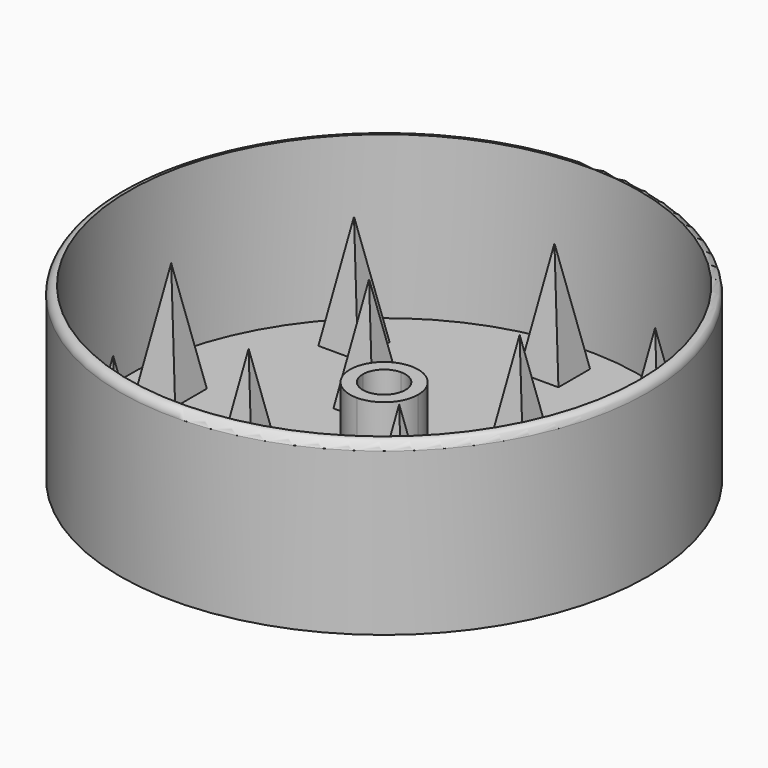
from build123d import *

# Parameters (mm, degrees)
F0_R     = 31
F0_R_2   = 30
F0_W     = 5
F0_H     = 5
F1_DEPTH = 1
F2_DEPTH = 20
F3_DEPTH = 10
F4_DEPTH = 15
F4_TAPER = 10
F5_R     = 0.99999
F6_DEPTH = 5


# Not quite as in the source:
# - a fillet or chamfer is up to 0.001 mm smaller than in the source, because OpenCascade refuses the exact size


with BuildPart() as f1:
    # F0 (on Top) → F1 (new body)
    with BuildSketch(Plane.XY):
        Circle(F0_R)
        Circle(F0_R_2, mode=Mode.SUBTRACT)
        Circle(F0_R_2)
        with Locations((-17.6776695297, -17.6776695297)):
            Rectangle(F0_W, F0_H, mode=Mode.SUBTRACT)
        Polygon((-2.5, -22.5), (0, -22.5), (2.5, -22.5), (2.5, -27.5), (-2.5, -27.5), align=None, mode=Mode.SUBTRACT)
        with Locations((17.6776695297, -17.6776695297)):
            Rectangle(F0_W, F0_H, mode=Mode.SUBTRACT)
        Polygon((-22.5, 2.5), (-22.5, 0), (-22.5, -2.5), (-27.5, -2.5), (-27.5, 2.5), align=None, mode=Mode.SUBTRACT)
        with Locations((-17.6776695297, 17.6776695297)):
            Rectangle(F0_W, F0_H, mode=Mode.SUBTRACT)
        with BuildLine():
            ThreePointArc((-15.1776695297, 15.1776695297), (-8.2140955588, 19.8305809006), (0, 21.4644660941))
            ThreePointArc((0, 21.4644660941), (8.2140955588, 19.8305809006), (15.1776695297, 15.1776695297))
            ThreePointArc((15.1776695297, 15.1776695297), (19.8305809006, 8.2140955588), (21.4644660941, 0))
            ThreePointArc((21.4644660941, 0), (19.8305809006, -8.2140955588), (15.1776695297, -15.1776695297))
            ThreePointArc((15.1776695297, -15.1776695297), (8.2140955588, -19.8305809006), (0, -21.4644660941))
            ThreePointArc((0, -21.4644660941), (-8.2140955588, -19.8305809006), (-15.1776695297, -15.1776695297))
            ThreePointArc((-15.1776695297, -15.1776695297), (-19.8305809006, -8.2140955588), (-21.4644660941, 0))
            ThreePointArc((-21.4644660941, 0), (-19.8305809006, 8.2140955588), (-15.1776695297, 15.1776695297))
        make_face(mode=Mode.SUBTRACT)
        Polygon((22.5, -2.5), (22.5, 0), (22.5, 2.5), (27.5, 2.5), (27.5, -2.5), align=None, mode=Mode.SUBTRACT)
        Polygon((2.5, 22.5), (0, 22.5), (-2.5, 22.5), (-2.5, 27.5), (2.5, 27.5), align=None, mode=Mode.SUBTRACT)
        with Locations((17.6776695297, 17.6776695297)):
            Rectangle(F0_W, F0_H, mode=Mode.SUBTRACT)
        with BuildLine():
            Line((0, 21.4644660941), (0, 12.5))
            ThreePointArc((0, 12.5), (3.2848701936, 12.0606644847), (6.3388347648, 10.7735404498))
            Line((6.3388347648, 10.7735404498), (6.3388347648, 11.3388347648))
            Line((6.3388347648, 11.3388347648), (11.3388347648, 11.3388347648))
            Line((11.3388347648, 11.3388347648), (15.1776695297, 15.1776695297))
            ThreePointArc((15.1776695297, 15.1776695297), (8.2140955588, 19.8305809006), (0, 21.4644660941))
        make_face()
        with BuildLine():
            ThreePointArc((10.7735404498, 6.3388347648), (12.0606644847, 3.2848701936), (12.5, 0))
            Line((12.5, 0), (21.4644660941, 0))
            ThreePointArc((21.4644660941, 0), (19.8305809006, 8.2140955588), (15.1776695297, 15.1776695297))
            Line((15.1776695297, 15.1776695297), (11.3388347648, 11.3388347648))
            Line((11.3388347648, 11.3388347648), (11.3388347648, 6.3388347648))
            Line((11.3388347648, 6.3388347648), (10.7735404498, 6.3388347648))
        make_face()
        with BuildLine():
            ThreePointArc((6.3388347648, -10.7735404498), (3.2848701936, -12.0606644847), (0, -12.5))
            Line((0, -12.5), (0, -21.4644660941))
            ThreePointArc((0, -21.4644660941), (8.2140955588, -19.8305809006), (15.1776695297, -15.1776695297))
            ThreePointArc((15.1776695297, -15.1776695297), (19.8305809006, -8.2140955588), (21.4644660941, 0))
            Line((21.4644660941, 0), (12.5, 0))
            ThreePointArc((12.5, 0), (12.0606644847, -3.2848701936), (10.7735404498, -6.3388347648))
            Line((10.7735404498, -6.3388347648), (11.3388347648, -6.3388347648))
            Line((11.3388347648, -6.3388347648), (11.3388347648, -11.3388347648))
            Line((11.3388347648, -11.3388347648), (6.3388347648, -11.3388347648))
            Line((6.3388347648, -11.3388347648), (6.3388347648, -10.7735404498))
        make_face()
        with BuildLine():
            Line((0, -21.4644660941), (0, -12.5))
            ThreePointArc((0, -12.5), (-3.2848701936, -12.0606644847), (-6.3388347648, -10.7735404498))
            Line((-6.3388347648, -10.7735404498), (-6.3388347648, -11.3388347648))
            Line((-6.3388347648, -11.3388347648), (-11.3388347648, -11.3388347648))
            Line((-11.3388347648, -11.3388347648), (-11.3388347648, -6.3388347648))
            Line((-11.3388347648, -6.3388347648), (-10.7735404498, -6.3388347648))
            ThreePointArc((-10.7735404498, -6.3388347648), (-12.0606644847, -3.2848701936), (-12.5, 0))
            Line((-12.5, 0), (-21.4644660941, 0))
            ThreePointArc((-21.4644660941, 0), (-19.8305809006, -8.2140955588), (-15.1776695297, -15.1776695297))
            ThreePointArc((-15.1776695297, -15.1776695297), (-8.2140955588, -19.8305809006), (0, -21.4644660941))
        make_face()
        with BuildLine():
            ThreePointArc((-6.3388347648, 10.7735404498), (-3.2848701936, 12.0606644847), (0, 12.5))
            Line((0, 12.5), (0, 21.4644660941))
            ThreePointArc((0, 21.4644660941), (-8.2140955588, 19.8305809006), (-15.1776695297, 15.1776695297))
            ThreePointArc((-15.1776695297, 15.1776695297), (-19.8305809006, 8.2140955588), (-21.4644660941, 0))
            Line((-21.4644660941, 0), (-12.5, 0))
            ThreePointArc((-12.5, 0), (-12.0606644847, 3.2848701936), (-10.7735404498, 6.3388347648))
            Line((-10.7735404498, 6.3388347648), (-11.3388347648, 6.3388347648))
            Line((-11.3388347648, 6.3388347648), (-11.3388347648, 11.3388347648))
            Line((-11.3388347648, 11.3388347648), (-6.3388347648, 11.3388347648))
            Line((-6.3388347648, 11.3388347648), (-6.3388347648, 10.7735404498))
        make_face()
        with BuildLine():
            Line((0, 12.5), (0, 4))
            ThreePointArc((0, 4), (1.5307337295, 3.69551813), (2.8284271247, 2.8284271247))
            Line((2.8284271247, 2.8284271247), (6.3388347648, 6.3388347648))
            Line((6.3388347648, 6.3388347648), (6.3388347648, 10.7735404498))
            ThreePointArc((6.3388347648, 10.7735404498), (3.2848701936, 12.0606644847), (0, 12.5))
        make_face()
        with BuildLine():
            ThreePointArc((-4, 0), (-2.8284271247, 2.8284271247), (0, 4))
            Line((0, 4), (0, 12.5))
            ThreePointArc((0, 12.5), (-3.2848701936, 12.0606644847), (-6.3388347648, 10.7735404498))
            Line((-6.3388347648, 10.7735404498), (-6.3388347648, 6.3388347648))
            Line((-6.3388347648, 6.3388347648), (-10.7735404498, 6.3388347648))
            ThreePointArc((-10.7735404498, 6.3388347648), (-12.0606644847, 3.2848701936), (-12.5, 0))
            Line((-12.5, 0), (-4, 0))
        make_face()
        with BuildLine():
            ThreePointArc((2.8284271247, 2.8284271247), (3.69551813, 1.5307337295), (4, 0))
            Line((4, 0), (12.5, 0))
            ThreePointArc((12.5, 0), (12.0606644847, 3.2848701936), (10.7735404498, 6.3388347648))
            Line((10.7735404498, 6.3388347648), (6.3388347648, 6.3388347648))
            Line((6.3388347648, 6.3388347648), (2.8284271247, 2.8284271247))
        make_face()
        with BuildLine():
            ThreePointArc((4, 0), (2.8284271247, -2.8284271247), (0, -4))
            Line((0, -4), (0, -12.5))
            ThreePointArc((0, -12.5), (3.2848701936, -12.0606644847), (6.3388347648, -10.7735404498))
            Line((6.3388347648, -10.7735404498), (6.3388347648, -6.3388347648))
            Line((6.3388347648, -6.3388347648), (10.7735404498, -6.3388347648))
            ThreePointArc((10.7735404498, -6.3388347648), (12.0606644847, -3.2848701936), (12.5, 0))
            Line((12.5, 0), (4, 0))
        make_face()
        with BuildLine():
            Line((0, -12.5), (0, -4))
            ThreePointArc((0, -4), (-2.8284271247, -2.8284271247), (-4, 0))
            Line((-4, 0), (-12.5, 0))
            ThreePointArc((-12.5, 0), (-12.0606644847, -3.2848701936), (-10.7735404498, -6.3388347648))
            Line((-10.7735404498, -6.3388347648), (-6.3388347648, -6.3388347648))
            Line((-6.3388347648, -6.3388347648), (-6.3388347648, -10.7735404498))
            ThreePointArc((-6.3388347648, -10.7735404498), (-3.2848701936, -12.0606644847), (0, -12.5))
        make_face()
        Polygon((22.5, 2.5), (25, 0), (27.5, 2.5), align=None)
        Polygon((27.5, 2.5), (25, 0), (27.5, -2.5), align=None)
        Polygon((27.5, -2.5), (25, 0), (22.5, -2.5), align=None)
        Polygon((25, 0), (22.5, 0), (22.5, -2.5), align=None)
        Polygon((22.5, 2.5), (22.5, 0), (25, 0), align=None)
        Polygon((17.6776695297, 17.6776695297), (15.1776695297, 15.1776695297), (20.1776695297, 15.1776695297), align=None)
        Polygon((15.1776695297, 20.1776695297), (17.6776695297, 17.6776695297), (20.1776695297, 20.1776695297), align=None)
        Polygon((20.1776695297, 20.1776695297), (17.6776695297, 17.6776695297), (20.1776695297, 15.1776695297), align=None)
        Polygon((15.1776695297, 20.1776695297), (15.1776695297, 15.1776695297), (17.6776695297, 17.6776695297), align=None)
        Polygon((-2.5, 27.5), (0, 25), (2.5, 27.5), align=None)
        Polygon((2.5, 27.5), (0, 25), (2.5, 22.5), align=None)
        Polygon((-2.5, 22.5), (0, 22.5), (0, 25), align=None)
        Polygon((0, 25), (0, 22.5), (2.5, 22.5), align=None)
        Polygon((-2.5, 22.5), (0, 25), (-2.5, 27.5), align=None)
        Polygon((-17.6776695297, 17.6776695297), (-15.1776695297, 20.1776695297), (-20.1776695297, 20.1776695297), align=None)
        Polygon((-17.6776695297, 17.6776695297), (-15.1776695297, 15.1776695297), (-15.1776695297, 20.1776695297), align=None)
        Polygon((-20.1776695297, 15.1776695297), (-15.1776695297, 15.1776695297), (-17.6776695297, 17.6776695297), align=None)
        Polygon((-20.1776695297, 20.1776695297), (-20.1776695297, 15.1776695297), (-17.6776695297, 17.6776695297), align=None)
        Polygon((-8.8388347762, 8.8388347535), (-6.3388347648, 11.3388347648), (-11.3388347648, 11.3388347648), align=None)
        Polygon((-11.3388347648, 6.3388347648), (-8.8388347762, 8.8388347535), (-11.3388347648, 11.3388347648), align=None)
        with BuildLine():
            ThreePointArc((-8.8388347762, 8.8388347535), (-9.8855356702, 7.650240814), (-10.7735404498, 6.3388347648))
            Line((-10.7735404498, 6.3388347648), (-6.3388347648, 6.3388347648))
            Line((-6.3388347648, 6.3388347648), (-8.8388347648, 8.8388347648))
        make_face()
        with BuildLine():
            Line((-6.3388347648, 6.3388347648), (-6.3388347648, 10.7735404498))
            ThreePointArc((-6.3388347648, 10.7735404498), (-7.6502408267, 9.8855356604), (-8.8388347762, 8.8388347535))
            Line((-8.8388347648, 8.8388347648), (-6.3388347648, 6.3388347648))
        make_face()
        with BuildLine():
            Line((6.3388347648, 10.7735404498), (6.3388347648, 6.3388347648))
            Line((6.3388347648, 6.3388347648), (8.8388347648, 8.8388347648))
            ThreePointArc((8.8388347535, 8.8388347762), (7.650240814, 9.8855356702), (6.3388347648, 10.7735404498))
        make_face()
        Polygon((6.3388347648, 11.3388347648), (8.8388347535, 8.8388347762), (11.3388347648, 11.3388347648), align=None)
        Polygon((11.3388347648, 11.3388347648), (8.8388347648, 8.8388347648), (11.3388347648, 6.3388347648), align=None)
        with BuildLine():
            Line((8.8388347648, 8.8388347648), (6.3388347648, 6.3388347648))
            Line((6.3388347648, 6.3388347648), (10.7735404498, 6.3388347648))
            ThreePointArc((10.7735404498, 6.3388347648), (9.8855356604, 7.6502408267), (8.8388347535, 8.8388347762))
        make_face()
        with BuildLine():
            ThreePointArc((8.8388347578, -8.8388347719), (9.8855356623, -7.6502408243), (10.7735404498, -6.3388347648))
            Line((10.7735404498, -6.3388347648), (6.3388347648, -6.3388347648))
            Line((6.3388347648, -6.3388347648), (8.8388347648, -8.8388347648))
        make_face()
        Polygon((11.3388347648, -6.3388347648), (8.8388347578, -8.8388347719), (11.3388347648, -11.3388347648), align=None)
        Polygon((8.8388347578, -8.8388347719), (6.3388347648, -11.3388347648), (11.3388347648, -11.3388347648), align=None)
        with BuildLine():
            Line((6.3388347648, -6.3388347648), (6.3388347648, -10.7735404498))
            ThreePointArc((6.3388347648, -10.7735404498), (7.6502408164, -9.8855356684), (8.8388347578, -8.8388347719))
            Line((8.8388347648, -8.8388347648), (6.3388347648, -6.3388347648))
        make_face()
        with BuildLine():
            Line((-6.3388347648, -6.3388347648), (-10.7735404498, -6.3388347648))
            ThreePointArc((-10.7735404498, -6.3388347648), (-9.8855356524, -7.650240837), (-8.838834735, -8.8388347946))
            Line((-8.8388347648, -8.8388347648), (-6.3388347648, -6.3388347648))
        make_face()
        with BuildLine():
            ThreePointArc((-8.838834735, -8.8388347946), (-7.6502408037, -9.8855356782), (-6.3388347648, -10.7735404498))
            Line((-6.3388347648, -10.7735404498), (-6.3388347648, -6.3388347648))
            Line((-6.3388347648, -6.3388347648), (-8.8388347648, -8.8388347648))
        make_face()
        Polygon((-11.3388347648, -11.3388347648), (-6.3388347648, -11.3388347648), (-8.838834735, -8.8388347946), align=None)
        Polygon((-27.5, 2.5), (-25, 0), (-22.5, 2.5), align=None)
        Polygon((-25, 0), (-22.5, 0), (-22.5, 2.5), align=None)
        Polygon((-22.5, -2.5), (-22.5, 0), (-25, 0), align=None)
        Polygon((-22.5, -2.5), (-25, 0), (-27.5, -2.5), align=None)
        Polygon((-27.5, -2.5), (-25, 0), (-27.5, 2.5), align=None)
        with BuildLine():
            ThreePointArc((-2.5, 0), (-1.767766953, 1.767766953), (0, 2.5))
            Line((0, 2.5), (0, 4))
            ThreePointArc((0, 4), (-2.8284271247, 2.8284271247), (-4, 0))
            Line((-4, 0), (-2.5, 0))
        make_face()
        with BuildLine():
            ThreePointArc((2.5, 0), (1.767766953, -1.767766953), (0, -2.5))
            Line((0, -2.5), (0, -4))
            ThreePointArc((0, -4), (2.8284271247, -2.8284271247), (4, 0))
            Line((4, 0), (2.5, 0))
        make_face()
        with BuildLine():
            Line((0, -4), (0, -2.5))
            ThreePointArc((0, -2.5), (-1.767766953, -1.767766953), (-2.5, 0))
            Line((-2.5, 0), (-4, 0))
            ThreePointArc((-4, 0), (-2.8284271247, -2.8284271247), (0, -4))
        make_face()
        with BuildLine():
            ThreePointArc((1.767766953, 1.767766953), (2.3096988313, 0.9567085809), (2.5, 0))
            Line((2.5, 0), (4, 0))
            ThreePointArc((4, 0), (3.69551813, 1.5307337295), (2.8284271247, 2.8284271247))
            Line((2.8284271247, 2.8284271247), (1.767766953, 1.767766953))
        make_face()
        with BuildLine():
            Line((0, 4), (0, 2.5))
            ThreePointArc((0, 2.5), (0.9567085809, 2.3096988313), (1.767766953, 1.767766953))
            Line((1.767766953, 1.767766953), (2.8284271247, 2.8284271247))
            ThreePointArc((2.8284271247, 2.8284271247), (1.5307337295, 3.69551813), (0, 4))
        make_face()
        Polygon((-11.3388347648, -11.3388347648), (-8.8388347648, -8.8388347648), (-11.3388347648, -6.3388347648), align=None)
        Polygon((-17.6776695297, -17.6776695297), (-15.1776695297, -15.1776695297), (-20.1776695297, -15.1776695297), align=None)
        Polygon((-15.1776695297, -20.1776695297), (-15.1776695297, -15.1776695297), (-17.6776695297, -17.6776695297), align=None)
        Polygon((-20.1776695297, -20.1776695297), (-15.1776695297, -20.1776695297), (-17.6776695297, -17.6776695297), align=None)
        Polygon((-17.6776695297, -17.6776695297), (-20.1776695297, -15.1776695297), (-20.1776695297, -20.1776695297), align=None)
        Polygon((20.1776695297, -15.1776695297), (15.1776695297, -15.1776695297), (17.6776695297, -17.6776695297), align=None)
        Polygon((20.1776695297, -20.1776695297), (20.1776695297, -15.1776695297), (17.6776695297, -17.6776695297), align=None)
        Polygon((17.6776695297, -17.6776695297), (15.1776695297, -20.1776695297), (20.1776695297, -20.1776695297), align=None)
        Polygon((17.6776695297, -17.6776695297), (15.1776695297, -15.1776695297), (15.1776695297, -20.1776695297), align=None)
        Polygon((2.5, -22.5), (0, -25), (2.5, -27.5), align=None)
        Polygon((2.5, -27.5), (0, -25), (-2.5, -27.5), align=None)
        Polygon((-2.5, -27.5), (0, -25), (-2.5, -22.5), align=None)
        Polygon((0, -25), (0, -22.5), (-2.5, -22.5), align=None)
        Polygon((2.5, -22.5), (0, -22.5), (0, -25), align=None)
        with BuildLine():
            Line((11.3388347648, -6.3388347648), (10.7735404498, -6.3388347648))
            ThreePointArc((10.7735404498, -6.3388347648), (9.8855356623, -7.6502408243), (8.8388347578, -8.8388347719))
            Line((8.8388347578, -8.8388347719), (11.3388347648, -6.3388347648))
        make_face()
        with BuildLine():
            ThreePointArc((8.8388347578, -8.8388347719), (7.6502408164, -9.8855356684), (6.3388347648, -10.7735404498))
            Line((6.3388347648, -10.7735404498), (6.3388347648, -11.3388347648))
            Line((6.3388347648, -11.3388347648), (8.8388347578, -8.8388347719))
        make_face()
        with BuildLine():
            Line((-6.3388347648, -11.3388347648), (-6.3388347648, -10.7735404498))
            ThreePointArc((-6.3388347648, -10.7735404498), (-7.6502408037, -9.8855356782), (-8.838834735, -8.8388347946))
            Line((-8.838834735, -8.8388347946), (-6.3388347648, -11.3388347648))
        make_face()
        with BuildLine():
            ThreePointArc((-8.838834735, -8.8388347946), (-9.8855356524, -7.650240837), (-10.7735404498, -6.3388347648))
            Line((-10.7735404498, -6.3388347648), (-11.3388347648, -6.3388347648))
            Line((-11.3388347648, -6.3388347648), (-8.838834735, -8.8388347946))
        make_face()
        with BuildLine():
            ThreePointArc((8.8388347535, 8.8388347762), (9.8855356604, 7.6502408267), (10.7735404498, 6.3388347648))
            Line((10.7735404498, 6.3388347648), (11.3388347648, 6.3388347648))
            Line((11.3388347648, 6.3388347648), (8.8388347535, 8.8388347762))
        make_face()
        with BuildLine():
            Line((6.3388347648, 11.3388347648), (6.3388347648, 10.7735404498))
            ThreePointArc((6.3388347648, 10.7735404498), (7.650240814, 9.8855356702), (8.8388347535, 8.8388347762))
            Line((8.8388347535, 8.8388347762), (6.3388347648, 11.3388347648))
        make_face()
        with BuildLine():
            ThreePointArc((-8.8388347762, 8.8388347535), (-7.6502408267, 9.8855356604), (-6.3388347648, 10.7735404498))
            Line((-6.3388347648, 10.7735404498), (-6.3388347648, 11.3388347648))
            Line((-6.3388347648, 11.3388347648), (-8.8388347762, 8.8388347535))
        make_face()
        with BuildLine():
            Line((-11.3388347648, 6.3388347648), (-10.7735404498, 6.3388347648))
            ThreePointArc((-10.7735404498, 6.3388347648), (-9.8855356702, 7.650240814), (-8.8388347762, 8.8388347535))
            Line((-8.8388347762, 8.8388347535), (-11.3388347648, 6.3388347648))
        make_face()
        with BuildLine():
            Line((0, 2.5), (0, 0))
            Line((0, 0), (1.767766953, 1.767766953))
            ThreePointArc((1.767766953, 1.767766953), (0.9567085809, 2.3096988313), (0, 2.5))
        make_face()
        with BuildLine():
            Line((1.767766953, 1.767766953), (0, 0))
            Line((0, 0), (2.5, 0))
            ThreePointArc((2.5, 0), (2.3096988313, 0.9567085809), (1.767766953, 1.767766953))
        make_face()
        with BuildLine():
            Line((2.5, 0), (0, 0))
            Line((0, 0), (0, -2.5))
            ThreePointArc((0, -2.5), (1.767766953, -1.767766953), (2.5, 0))
        make_face()
        with BuildLine():
            Line((0, -2.5), (0, 0))
            Line((0, 0), (-2.5, 0))
            ThreePointArc((-2.5, 0), (-1.767766953, -1.767766953), (0, -2.5))
        make_face()
        with BuildLine():
            Line((-2.5, 0), (0, 0))
            Line((0, 0), (0, 2.5))
            ThreePointArc((0, 2.5), (-1.767766953, 1.767766953), (-2.5, 0))
        make_face()
    extrude(amount=F1_DEPTH)

    # F0 (on Top) → F2 (join)
    with BuildSketch(Plane.XY):
        Circle(F0_R)
        Circle(F0_R_2, mode=Mode.SUBTRACT)
    extrude(amount=F2_DEPTH)

    # F0 (on Top) → F3 (join)
    with BuildSketch(Plane.XY):
        with BuildLine():
            ThreePointArc((2.5, 0), (1.767766953, -1.767766953), (0, -2.5))
            Line((0, -2.5), (0, -4))
            ThreePointArc((0, -4), (2.8284271247, -2.8284271247), (4, 0))
            Line((4, 0), (2.5, 0))
        make_face()
        with BuildLine():
            ThreePointArc((1.767766953, 1.767766953), (2.3096988313, 0.9567085809), (2.5, 0))
            Line((2.5, 0), (4, 0))
            ThreePointArc((4, 0), (3.69551813, 1.5307337295), (2.8284271247, 2.8284271247))
            Line((2.8284271247, 2.8284271247), (1.767766953, 1.767766953))
        make_face()
        with BuildLine():
            Line((0, 4), (0, 2.5))
            ThreePointArc((0, 2.5), (0.9567085809, 2.3096988313), (1.767766953, 1.767766953))
            Line((1.767766953, 1.767766953), (2.8284271247, 2.8284271247))
            ThreePointArc((2.8284271247, 2.8284271247), (1.5307337295, 3.69551813), (0, 4))
        make_face()
        with BuildLine():
            ThreePointArc((-2.5, 0), (-1.767766953, 1.767766953), (0, 2.5))
            Line((0, 2.5), (0, 4))
            ThreePointArc((0, 4), (-2.8284271247, 2.8284271247), (-4, 0))
            Line((-4, 0), (-2.5, 0))
        make_face()
        with BuildLine():
            Line((0, -4), (0, -2.5))
            ThreePointArc((0, -2.5), (-1.767766953, -1.767766953), (-2.5, 0))
            Line((-2.5, 0), (-4, 0))
            ThreePointArc((-4, 0), (-2.8284271247, -2.8284271247), (0, -4))
        make_face()
    extrude(amount=F3_DEPTH)

    # F0 (on Top) → F4 (join)
    with BuildSketch(Plane.XY):
        Polygon((2.5, -27.5), (0, -25), (-2.5, -27.5), align=None)
        Polygon((2.5, -22.5), (0, -25), (2.5, -27.5), align=None)
        Polygon((2.5, -22.5), (0, -22.5), (0, -25), align=None)
        Polygon((0, -25), (0, -22.5), (-2.5, -22.5), align=None)
        Polygon((-2.5, -27.5), (0, -25), (-2.5, -22.5), align=None)
        Polygon((17.6776695297, -17.6776695297), (15.1776695297, -15.1776695297), (15.1776695297, -20.1776695297), align=None)
        Polygon((17.6776695297, -17.6776695297), (15.1776695297, -20.1776695297), (20.1776695297, -20.1776695297), align=None)
        Polygon((20.1776695297, -20.1776695297), (20.1776695297, -15.1776695297), (17.6776695297, -17.6776695297), align=None)
        Polygon((20.1776695297, -15.1776695297), (15.1776695297, -15.1776695297), (17.6776695297, -17.6776695297), align=None)
        Polygon((8.8388347578, -8.8388347719), (6.3388347648, -11.3388347648), (11.3388347648, -11.3388347648), align=None)
        with BuildLine():
            Line((6.3388347648, -6.3388347648), (6.3388347648, -10.7735404498))
            ThreePointArc((6.3388347648, -10.7735404498), (7.6502408164, -9.8855356684), (8.8388347578, -8.8388347719))
            Line((8.8388347648, -8.8388347648), (6.3388347648, -6.3388347648))
        make_face()
        Polygon((11.3388347648, -6.3388347648), (8.8388347578, -8.8388347719), (11.3388347648, -11.3388347648), align=None)
        with BuildLine():
            ThreePointArc((8.8388347578, -8.8388347719), (9.8855356623, -7.6502408243), (10.7735404498, -6.3388347648))
            Line((10.7735404498, -6.3388347648), (6.3388347648, -6.3388347648))
            Line((6.3388347648, -6.3388347648), (8.8388347648, -8.8388347648))
        make_face()
        with BuildLine():
            Line((11.3388347648, -6.3388347648), (10.7735404498, -6.3388347648))
            ThreePointArc((10.7735404498, -6.3388347648), (9.8855356623, -7.6502408243), (8.8388347578, -8.8388347719))
            Line((8.8388347578, -8.8388347719), (11.3388347648, -6.3388347648))
        make_face()
        with BuildLine():
            ThreePointArc((8.8388347578, -8.8388347719), (7.6502408164, -9.8855356684), (6.3388347648, -10.7735404498))
            Line((6.3388347648, -10.7735404498), (6.3388347648, -11.3388347648))
            Line((6.3388347648, -11.3388347648), (8.8388347578, -8.8388347719))
        make_face()
        Polygon((-11.3388347648, -11.3388347648), (-6.3388347648, -11.3388347648), (-8.838834735, -8.8388347946), align=None)
        with BuildLine():
            ThreePointArc((-8.838834735, -8.8388347946), (-7.6502408037, -9.8855356782), (-6.3388347648, -10.7735404498))
            Line((-6.3388347648, -10.7735404498), (-6.3388347648, -6.3388347648))
            Line((-6.3388347648, -6.3388347648), (-8.8388347648, -8.8388347648))
        make_face()
        with BuildLine():
            Line((-6.3388347648, -6.3388347648), (-10.7735404498, -6.3388347648))
            ThreePointArc((-10.7735404498, -6.3388347648), (-9.8855356524, -7.650240837), (-8.838834735, -8.8388347946))
            Line((-8.8388347648, -8.8388347648), (-6.3388347648, -6.3388347648))
        make_face()
        Polygon((-11.3388347648, -11.3388347648), (-8.8388347648, -8.8388347648), (-11.3388347648, -6.3388347648), align=None)
        with BuildLine():
            Line((-6.3388347648, -11.3388347648), (-6.3388347648, -10.7735404498))
            ThreePointArc((-6.3388347648, -10.7735404498), (-7.6502408037, -9.8855356782), (-8.838834735, -8.8388347946))
            Line((-8.838834735, -8.8388347946), (-6.3388347648, -11.3388347648))
        make_face()
        with BuildLine():
            ThreePointArc((-8.838834735, -8.8388347946), (-9.8855356524, -7.650240837), (-10.7735404498, -6.3388347648))
            Line((-10.7735404498, -6.3388347648), (-11.3388347648, -6.3388347648))
            Line((-11.3388347648, -6.3388347648), (-8.838834735, -8.8388347946))
        make_face()
        Polygon((-15.1776695297, -20.1776695297), (-15.1776695297, -15.1776695297), (-17.6776695297, -17.6776695297), align=None)
        Polygon((-20.1776695297, -20.1776695297), (-15.1776695297, -20.1776695297), (-17.6776695297, -17.6776695297), align=None)
        Polygon((-17.6776695297, -17.6776695297), (-20.1776695297, -15.1776695297), (-20.1776695297, -20.1776695297), align=None)
        Polygon((-17.6776695297, -17.6776695297), (-15.1776695297, -15.1776695297), (-20.1776695297, -15.1776695297), align=None)
        Polygon((-22.5, -2.5), (-25, 0), (-27.5, -2.5), align=None)
        Polygon((-22.5, -2.5), (-22.5, 0), (-25, 0), align=None)
        Polygon((-25, 0), (-22.5, 0), (-22.5, 2.5), align=None)
        Polygon((-27.5, 2.5), (-25, 0), (-22.5, 2.5), align=None)
        Polygon((-27.5, -2.5), (-25, 0), (-27.5, 2.5), align=None)
        Polygon((27.5, -2.5), (25, 0), (22.5, -2.5), align=None)
        Polygon((27.5, 2.5), (25, 0), (27.5, -2.5), align=None)
        Polygon((25, 0), (22.5, 0), (22.5, -2.5), align=None)
        Polygon((22.5, 2.5), (22.5, 0), (25, 0), align=None)
        Polygon((22.5, 2.5), (25, 0), (27.5, 2.5), align=None)
        with BuildLine():
            Line((6.3388347648, 10.7735404498), (6.3388347648, 6.3388347648))
            Line((6.3388347648, 6.3388347648), (8.8388347648, 8.8388347648))
            ThreePointArc((8.8388347535, 8.8388347762), (7.650240814, 9.8855356702), (6.3388347648, 10.7735404498))
        make_face()
        Polygon((11.3388347648, 11.3388347648), (8.8388347648, 8.8388347648), (11.3388347648, 6.3388347648), align=None)
        with BuildLine():
            Line((8.8388347648, 8.8388347648), (6.3388347648, 6.3388347648))
            Line((6.3388347648, 6.3388347648), (10.7735404498, 6.3388347648))
            ThreePointArc((10.7735404498, 6.3388347648), (9.8855356604, 7.6502408267), (8.8388347535, 8.8388347762))
        make_face()
        Polygon((6.3388347648, 11.3388347648), (8.8388347535, 8.8388347762), (11.3388347648, 11.3388347648), align=None)
        with BuildLine():
            ThreePointArc((8.8388347535, 8.8388347762), (9.8855356604, 7.6502408267), (10.7735404498, 6.3388347648))
            Line((10.7735404498, 6.3388347648), (11.3388347648, 6.3388347648))
            Line((11.3388347648, 6.3388347648), (8.8388347535, 8.8388347762))
        make_face()
        with BuildLine():
            Line((6.3388347648, 11.3388347648), (6.3388347648, 10.7735404498))
            ThreePointArc((6.3388347648, 10.7735404498), (7.650240814, 9.8855356702), (8.8388347535, 8.8388347762))
            Line((8.8388347535, 8.8388347762), (6.3388347648, 11.3388347648))
        make_face()
        with BuildLine():
            ThreePointArc((-8.8388347762, 8.8388347535), (-9.8855356702, 7.650240814), (-10.7735404498, 6.3388347648))
            Line((-10.7735404498, 6.3388347648), (-6.3388347648, 6.3388347648))
            Line((-6.3388347648, 6.3388347648), (-8.8388347648, 8.8388347648))
        make_face()
        with BuildLine():
            Line((-11.3388347648, 6.3388347648), (-10.7735404498, 6.3388347648))
            ThreePointArc((-10.7735404498, 6.3388347648), (-9.8855356702, 7.650240814), (-8.8388347762, 8.8388347535))
            Line((-8.8388347762, 8.8388347535), (-11.3388347648, 6.3388347648))
        make_face()
        Polygon((-11.3388347648, 6.3388347648), (-8.8388347762, 8.8388347535), (-11.3388347648, 11.3388347648), align=None)
        with BuildLine():
            Line((-6.3388347648, 6.3388347648), (-6.3388347648, 10.7735404498))
            ThreePointArc((-6.3388347648, 10.7735404498), (-7.6502408267, 9.8855356604), (-8.8388347762, 8.8388347535))
            Line((-8.8388347648, 8.8388347648), (-6.3388347648, 6.3388347648))
        make_face()
        Polygon((-8.8388347762, 8.8388347535), (-6.3388347648, 11.3388347648), (-11.3388347648, 11.3388347648), align=None)
        with BuildLine():
            ThreePointArc((-8.8388347762, 8.8388347535), (-7.6502408267, 9.8855356604), (-6.3388347648, 10.7735404498))
            Line((-6.3388347648, 10.7735404498), (-6.3388347648, 11.3388347648))
            Line((-6.3388347648, 11.3388347648), (-8.8388347762, 8.8388347535))
        make_face()
        Polygon((17.6776695297, 17.6776695297), (15.1776695297, 15.1776695297), (20.1776695297, 15.1776695297), align=None)
        Polygon((20.1776695297, 20.1776695297), (17.6776695297, 17.6776695297), (20.1776695297, 15.1776695297), align=None)
        Polygon((15.1776695297, 20.1776695297), (17.6776695297, 17.6776695297), (20.1776695297, 20.1776695297), align=None)
        Polygon((15.1776695297, 20.1776695297), (15.1776695297, 15.1776695297), (17.6776695297, 17.6776695297), align=None)
        Polygon((-20.1776695297, 15.1776695297), (-15.1776695297, 15.1776695297), (-17.6776695297, 17.6776695297), align=None)
        Polygon((-20.1776695297, 20.1776695297), (-20.1776695297, 15.1776695297), (-17.6776695297, 17.6776695297), align=None)
        Polygon((-17.6776695297, 17.6776695297), (-15.1776695297, 15.1776695297), (-15.1776695297, 20.1776695297), align=None)
        Polygon((-17.6776695297, 17.6776695297), (-15.1776695297, 20.1776695297), (-20.1776695297, 20.1776695297), align=None)
        Polygon((-2.5, 22.5), (0, 25), (-2.5, 27.5), align=None)
        Polygon((-2.5, 27.5), (0, 25), (2.5, 27.5), align=None)
        Polygon((2.5, 27.5), (0, 25), (2.5, 22.5), align=None)
        Polygon((0, 25), (0, 22.5), (2.5, 22.5), align=None)
        Polygon((-2.5, 22.5), (0, 22.5), (0, 25), align=None)
    extrude(amount=F4_DEPTH, taper=F4_TAPER)

    # F5 (radius 1 in the source; OpenCascade refuses exactly that, so slightly less here)
    f5_edges = [f1.edges().sort_by_distance(p)[0] for p in [
        (-31, 0, 20),
    ]]
    fillet(f5_edges, radius=F5_R)

    # F6 (add): a face of the model
    f6_faces = [f1.faces().sort_by_distance(p)[0] for p in [
        (0, 0, 1),
    ]]
    extrude(f6_faces, amount=F6_DEPTH)


solid = f1.part
